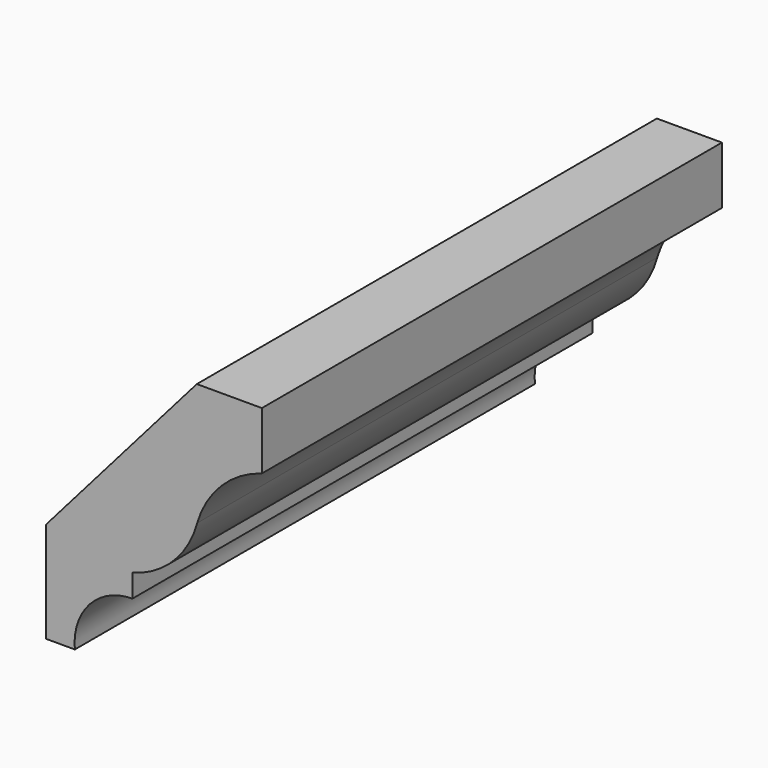
from build123d import *

# Parameters (mm, degrees)
F1_DEPTH = 127


# Not quite as in the source:
# - ends of sketch curves that miss each other by under 0.0002 mm in the source are joined


with BuildPart() as f1:
    # F0 (on Front) → F1 (new body)
    with BuildSketch(Plane.XZ):
        with BuildLine():
            Line((23.829137, 17.474692), (23.829137, 30.1835566))
            Line((23.829137, 30.1835566), (9.4594934, 30.1835566))
            Line((9.4594934, 30.1835566), (-23.8291116, -7.9430372))
            Line((-23.8291116, -7.9430372), (-23.8291116, -30.1835312))
            Line((-23.8291116, -30.1835312), (-17.474692, -30.1835312))
            ThreePointArc((-17.474692, -30.1835312), (-14.2269141432, -20.357689713), (-4.7658274, -16.1644838))
            Line((-4.7658274, -16.1644838), (-4.7658274, -11.120247))
            ThreePointArc((-4.7658274, -11.120247), (4.2916437043, -5.8802359043), (9.5316594554, 3.1772339438))
            ThreePointArc((9.5316594554, 3.1772339438), (14.8680934033, 12.1382706133), (23.829137, 17.474692))
        make_face()
    extrude(amount=-F1_DEPTH)


solid = f1.part
